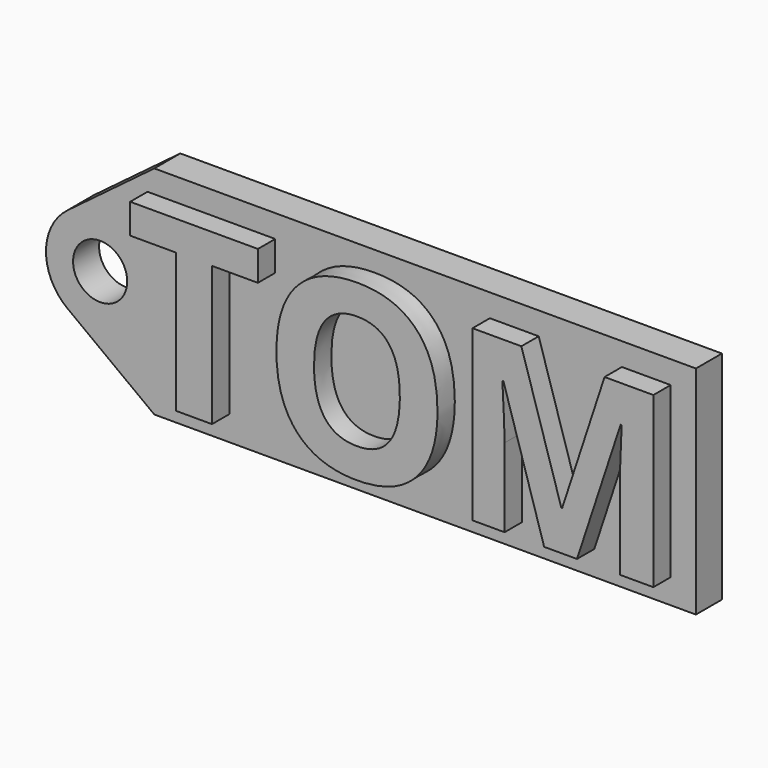
from build123d import *

# Parameters (mm, degrees)
F0_R         = 2.5
F1_DEPTH     = 3
F2_TEXT_SIZE = 21.8749997051
F3_DEPTH     = 2


# Not quite as in the source:
# - Text() gives the source's letters only with a copy of the font that has no kerning and outlines rounded to 1/6400 em; it was checked with that copy


with BuildPart() as f1:
    # F0 (on Front) → F1 (new body)
    with BuildSketch(Plane.XZ):
        with BuildLine():
            Line((-25, -10), (25, -10))
            Line((25, -10), (25, 10))
            Line((25, 10), (-25, 10))
            Line((-25, 10), (-33, 4))
            ThreePointArc((-33, 4), (-34.472135955, 2.2360679775), (-35, 0))
            ThreePointArc((-35, 0), (-34.472135955, -2.2360679775), (-33, -4))
            Line((-33, -4), (-25, -10))
        make_face()
        with Locations((-30, 0)):
            Circle(F0_R, mode=Mode.SUBTRACT)
    extrude(amount=F1_DEPTH)

    # F2 (on face) → F3 (join)
    with BuildSketch(Plane.XZ.offset(3)):
        with Locations((-26.0662510991, -7.7174999751)):
            Text('TOM', F2_TEXT_SIZE, font='Open Sans', font_style=FontStyle.BOLD, text_align=(TextAlign.LEFT, TextAlign.BOTTOM))
    extrude(amount=F3_DEPTH)


solid = f1.part
